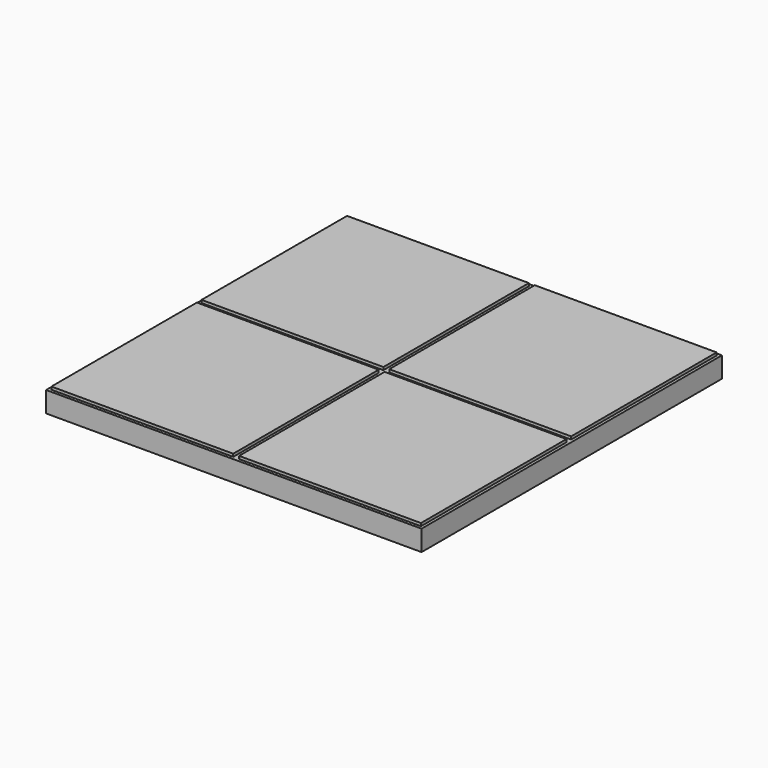
from build123d import *

# Parameters (mm, degrees)
F0_W     = 406.4
F0_H     = 406.4
F1_DEPTH = 25.4
F2_W     = 425.3633022308
F2_H     = 428.5580217838
F2_W_2   = 196.85
F2_H_2   = 196.85
F3_DEPTH = 3.048


# Not quite as in the source:
# - a feature names something its author has since deleted; it is built from what else it names


with BuildPart() as f1:
    # F0 (on Top) → F1 (new body)
    with BuildSketch(Plane.XY):
        Rectangle(F0_W, F0_H)
    extrude(amount=-F1_DEPTH)

    # F2 (on Top) → F3 (cut)
    with BuildSketch(Plane.XY):
        Rectangle(F2_W, F2_H)
        with Locations((-101.6, -101.6)):
            Rectangle(F2_W_2, F2_H_2, mode=Mode.SUBTRACT)
        with Locations((101.6, -101.6)):
            Rectangle(F2_W_2, F2_H_2, mode=Mode.SUBTRACT)
        with Locations((-101.6, 101.6)):
            Rectangle(F2_W_2, F2_H_2, mode=Mode.SUBTRACT)
        with Locations((101.6, 101.6)):
            Rectangle(F2_W_2, F2_H_2, mode=Mode.SUBTRACT)
    extrude(amount=-F3_DEPTH, mode=Mode.SUBTRACT)


solid = f1.part
